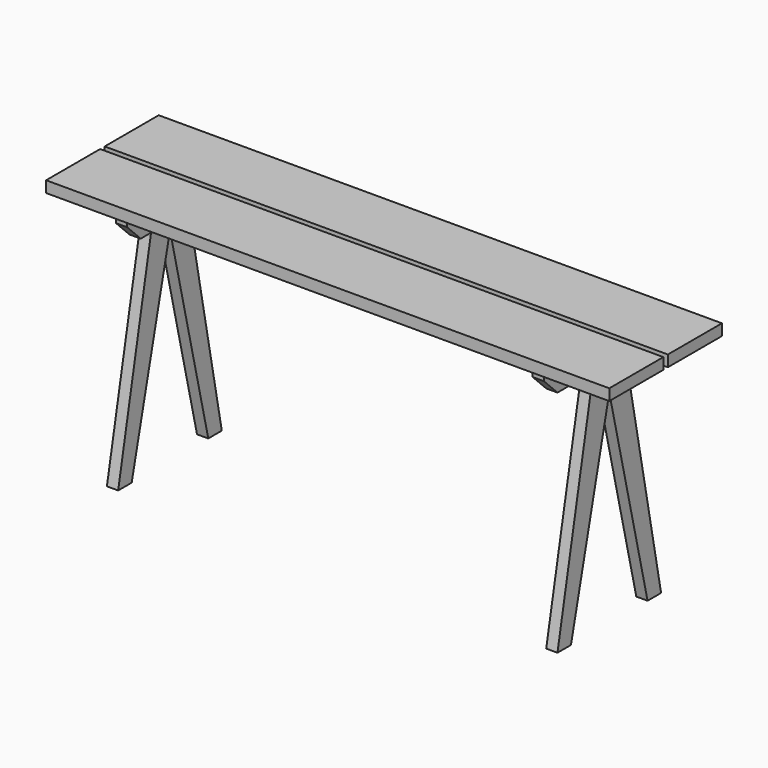
from build123d import *

# Parameters (mm, degrees)
F0_W      = 1000
F0_H      = 120
F1_DEPTH  = 20
F2_W      = 20
F2_H      = 40
F3_DEPTH  = 120
F5_START  = 380
F5_DEPTH  = 20
F6_START  = -380
F6_DEPTH  = 20
F7_SIZE   = 30
F7_2_SIZE = 30


with BuildPart() as f1:
    # F0 (on Top) → F1 (new body)
    with BuildSketch(Plane.XY):
        with Locations((0, 65)):
            Rectangle(F0_W, F0_H)
    extrude(amount=F1_DEPTH)


with BuildPart() as f1b:
    # F0 (on Top) → F1, piece 2 (new body)
    with BuildSketch(Plane.XY):
        with Locations((0, -65)):
            Rectangle(F0_W, F0_H)
    extrude(amount=F1_DEPTH)


with BuildPart() as f3:
    # F2 (on Front) → F3 (new body, symmetric)
    with BuildSketch(Plane.XZ):
        with Locations((-370, -20)):
            Rectangle(F2_W, F2_H)
    extrude(amount=F3_DEPTH, both=True)

    # F7
    f7_edges = [f3.edges().sort_by_distance(p)[0] for p in [
        (-370, -120, -40),
        (-370, 120, -40),
    ]]
    chamfer(f7_edges, length=F7_SIZE)


with BuildPart() as f3b:
    # F2 (on Front) → F3, piece 2 (new body, symmetric)
    with BuildSketch(Plane.XZ):
        with Locations((370, -20)):
            Rectangle(F2_W, F2_H)
    extrude(amount=F3_DEPTH, both=True)

    # F7#2
    f7_2_edges = [f3b.edges().sort_by_distance(p)[0] for p in [
        (370, -120, -40),
        (370, 120, -40),
    ]]
    chamfer(f7_2_edges, length=F7_2_SIZE)


with BuildPart() as f5:
    # F4 (on Right) → F5 (new body)
    with BuildSketch(Plane.YZ.offset(F5_START)):
        Polygon((30.9321093395, 0), (0, 0), (0, -70), (85, -430), (115, -430), align=None)
        Polygon((0, -70), (0, 0), (-30.9321093395, 0), (-115, -430), (-85, -430), align=None)
    extrude(amount=F5_DEPTH)


with BuildPart() as f6:
    # F4 (on Right) → F6 (new body)
    with BuildSketch(Plane.YZ.offset(F6_START)):
        Polygon((30.9321093395, 0), (0, 0), (0, -70), (85, -430), (115, -430), align=None)
        Polygon((0, -70), (0, 0), (-30.9321093395, 0), (-115, -430), (-85, -430), align=None)
    extrude(amount=-F6_DEPTH)


solid = Compound([f1.part, f1b.part, f3.part, f3b.part, f5.part, f6.part])
